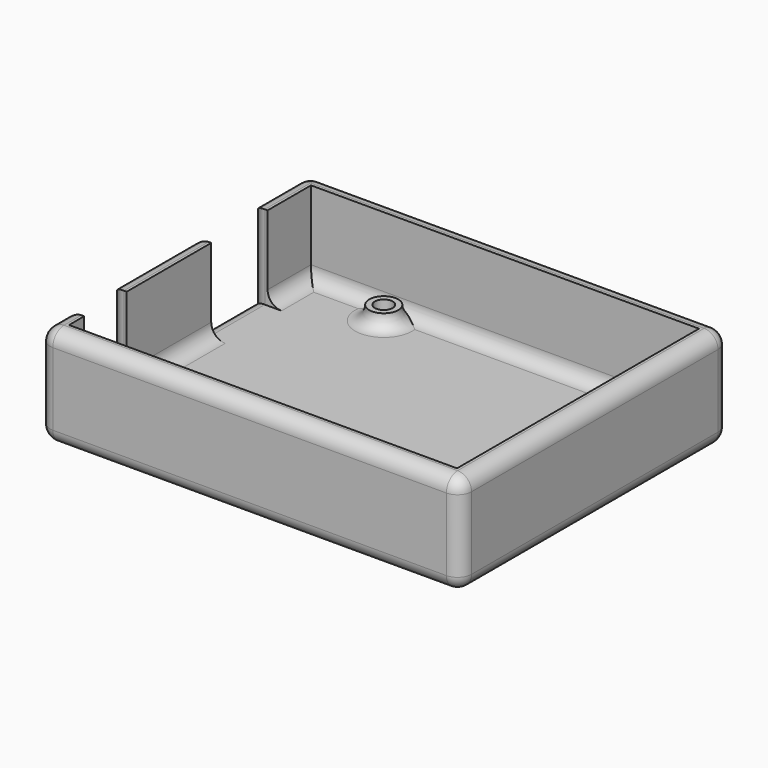
from build123d import *

# Parameters (mm, degrees)
F0_W          = 0.4
F0_H          = 0.3
F0_H_2        = 8.9
F0_W_2        = 9.5
F0_R          = 2.6
F0_W_3        = 10.3
F0_H_3        = 12
F0_W_4        = 3
F0_R_2        = 1.6
F0_H_4        = 18.9
F1_DEPTH      = 3
F2_DEPTH      = 15
F3_DEPTH      = 2.5
F4_T1_DEPTH   = 9.7
F4_T3_DEPTH   = 18.9
F4_T5_DEPTH   = 3.4
F4_T10_DEPTH  = 69.4
F4_S11_R      = 2.6
F4_T12_DEPTH  = 36
F4_T16_DEPTH  = 69.4
F4_S17_R      = 2.6
F4_T18_DEPTH  = 36
F4_T22_DEPTH  = 54.1
F4_S23_R      = 2.6
F4_T24_DEPTH  = 29
F4_S25_R      = 2.6
F4_T26_DEPTH  = 29
F4_T35_DEPTH  = 13
F4_T37_DEPTH  = 21.25
F4_T39_DEPTH  = 12.6
F4_T41_DEPTH  = 9.5
F4_T43_DEPTH  = 55.1
F4_T45_DEPTH  = 70.4
F4_T47_DEPTH  = 31.4
F4_T49_DEPTH  = 16.45
F4_T51_DEPTH  = 10.15
F4_S55_W      = 2.55
F4_S55_H      = 2.55
F4_T56_DEPTH  = 2.55
F4_S61_W      = 2.55
F4_S61_H      = 2.55
F4_T62_DEPTH  = 2.55
F4_S67_W      = 2.55
F4_S67_H      = 2.55
F4_T68_DEPTH  = 2.55
F4_S73_W      = 2.55
F4_S73_H      = 2.55
F4_T74_DEPTH  = 2.55
F4_S79_W      = 2.55
F4_S79_H      = 2.55
F4_T80_DEPTH  = 2.55
F4_S85_W      = 2.55
F4_S85_H      = 2.55
F4_T86_DEPTH  = 2.55
F4_S91_W      = 2.55
F4_S91_H      = 2.55
F4_T92_DEPTH  = 2.55
F4_S97_W      = 2.55
F4_S97_H      = 2.55
F4_T98_DEPTH  = 2.55
F4_T105_DEPTH = 15.75
F4_T109_DEPTH = 21.25
F4_T117_DEPTH = 18.85
F4_T121_DEPTH = 21.25
F4_T129_DEPTH = 21.25
F4_T134_DEPTH = 18.85
F4_T141_DEPTH = 21.25
F4_T146_DEPTH = 15.75


# Not quite as in the source:
# - a fillet or chamfer that OpenCascade refuses, or shapes differently, is made with other operations: its cross-section is extruded or revolved along the edge and cut away or added


with BuildPart() as f1:
    # F0 (on Top) → F1 (new body)
    with BuildSketch(Plane.XY):
        Polygon((-34.7, -27.05), (-34.7, -23.65), (-37.7, -23.65), (-37.7, -30.05), (37.7, -30.05), (37.7, 30.05), (-37.7, 30.05), (-37.7, 17.35), (-34.7, 17.35), (-34.7, 27.05), (34.7, 27.05), (34.7, -27.05), align=None)
        with Locations((-34.5, -14.3)):
            Rectangle(F0_W, F0_H)
        with Locations((-34.5, -18.9)):
            Rectangle(F0_W, F0_H_2)
        with Locations((-29.55, -18.9)):
            Rectangle(F0_W_2, F0_H_2)
        Polygon((-34.3, -26.65), (34.3, -26.65), (34.3, 26.65), (-34.3, 26.65), (-34.3, 17.35), (-23.7, 17.35), (-23.7, 4.75), (-34.3, 4.75), (-34.3, -14.15), (-24.5, -14.15), (-24.5, -23.65), (-34.3, -23.65), align=None)
        with Locations((-20.3, -23.85)):
            Circle(F0_R, mode=Mode.SUBTRACT)
        with Locations((31.6, -19.15)):
            Circle(F0_R, mode=Mode.SUBTRACT)
        with Locations((-19.2, 23.95)):
            Circle(F0_R, mode=Mode.SUBTRACT)
        with Locations((31.6, 8.75)):
            Circle(F0_R, mode=Mode.SUBTRACT)
        Polygon((34.3, 26.65), (34.3, -26.65), (-34.3, -26.65), (-34.3, -23.65), (-34.7, -23.65), (-34.7, -27.05), (34.7, -27.05), (34.7, 27.05), (-34.7, 27.05), (-34.7, 17.35), (-34.3, 17.35), (-34.3, 26.65), align=None)
        with Locations((-29.15, 11.05)):
            Rectangle(F0_W_3, F0_H_3)
        with Locations((-36.2, 11.05)):
            Rectangle(F0_W_4, F0_H_3)
        with Locations((-34.5, 11.05)):
            Rectangle(F0_W, F0_H_3)
        with Locations((-36.2, -18.9)):
            Rectangle(F0_W_4, F0_H_2)
        with Locations((-36.2, -14.3)):
            Rectangle(F0_W_4, F0_H)
        with Locations((-19.2, 23.95)):
            Circle(F0_R)
        with Locations((-19.2, 23.95)):
            Circle(F0_R_2, mode=Mode.SUBTRACT)
        with Locations((-20.3, -23.85)):
            Circle(F0_R)
        with Locations((-20.3, -23.85)):
            Circle(F0_R_2, mode=Mode.SUBTRACT)
        with Locations((31.6, -19.15)):
            Circle(F0_R)
        with Locations((31.6, -19.15)):
            Circle(F0_R_2, mode=Mode.SUBTRACT)
        with Locations((31.6, 8.75)):
            Circle(F0_R)
        with Locations((31.6, 8.75)):
            Circle(F0_R_2, mode=Mode.SUBTRACT)
        with Locations((-36.2, 4.9)):
            Rectangle(F0_W_4, F0_H)
        with Locations((-34.5, 4.9)):
            Rectangle(F0_W, F0_H)
        Polygon((-23.7, 17.35), (-34.3, 17.35), (-34.3, 17.05), (-24, 17.05), (-24, 5.05), (-34.3, 5.05), (-34.3, 4.75), (-23.7, 4.75), align=None)
        with Locations((-34.5, -4.7)):
            Rectangle(F0_W, F0_H_4)
        with Locations((-36.2, -4.7)):
            Rectangle(F0_W_4, F0_H_4)
        Polygon((-34.3, -23.35), (-34.3, -23.65), (-24.5, -23.65), (-24.5, -14.15), (-34.3, -14.15), (-34.3, -14.45), (-24.8, -14.45), (-24.8, -23.35), align=None)
        with Locations((-36.2, 17.2)):
            Rectangle(F0_W_4, F0_H)
        with Locations((-34.5, 17.2)):
            Rectangle(F0_W, F0_H)
        with Locations((-34.5, -23.5)):
            Rectangle(F0_W, F0_H)
        with Locations((-36.2, -23.5)):
            Rectangle(F0_W_4, F0_H)
    extrude(amount=-F1_DEPTH)

    # F0 (on Top) → F2 (join)
    with BuildSketch(Plane.XY):
        Polygon((-34.7, -27.05), (-34.7, -23.65), (-37.7, -23.65), (-37.7, -30.05), (37.7, -30.05), (37.7, 30.05), (-37.7, 30.05), (-37.7, 17.35), (-34.7, 17.35), (-34.7, 27.05), (34.7, 27.05), (34.7, -27.05), align=None)
        with Locations((-36.2, -4.7)):
            Rectangle(F0_W_4, F0_H_4)
    extrude(amount=F2_DEPTH)

    # F0 (on Top) → F3 (join)
    with BuildSketch(Plane.XY):
        with Locations((-20.3, -23.85)):
            Circle(F0_R)
        with Locations((-20.3, -23.85)):
            Circle(F0_R_2, mode=Mode.SUBTRACT)
        with Locations((-19.2, 23.95)):
            Circle(F0_R)
        with Locations((-19.2, 23.95)):
            Circle(F0_R_2, mode=Mode.SUBTRACT)
        with Locations((31.6, 8.75)):
            Circle(F0_R)
        with Locations((31.6, 8.75)):
            Circle(F0_R_2, mode=Mode.SUBTRACT)
        with Locations((31.6, -19.15)):
            Circle(F0_R)
        with Locations((31.6, -19.15)):
            Circle(F0_R_2, mode=Mode.SUBTRACT)
    extrude(amount=F3_DEPTH)

    # F4: fillet of radius 2.5 on 30 edges, made by hand

    # F4_s2 → F4_t1 (join)
    with BuildSketch(Plane.XZ.offset(-27.05)):
        with BuildLine():
            ThreePointArc((-34.7, 2.5), (-33.967766953, 0.732233047), (-32.2, 0))
            Line((-32.2, 0), (-34.7, 0))
            Line((-34.7, 0), (-34.7, 2.5))
        make_face()
    extrude(amount=F4_T1_DEPTH)

    # F4_s4 → F4_t3 (join)
    with BuildSketch(Plane.XZ.offset(-4.75)):
        with BuildLine():
            ThreePointArc((-32.2, 0), (-33.967766953, 0.732233047), (-34.7, 2.5))
            Line((-34.7, 2.5), (-34.7, 0))
            Line((-34.7, 0), (-32.2, 0))
        make_face()
    extrude(amount=F4_T3_DEPTH)

    # F4_s6 → F4_t5 (join)
    with BuildSketch(Plane.XZ.offset(23.65)):
        with BuildLine():
            ThreePointArc((-34.7, 2.5), (-33.967766953, 0.732233047), (-32.2, 0))
            Line((-32.2, 0), (-34.7, 0))
            Line((-34.7, 0), (-34.7, 2.5))
        make_face()
    extrude(amount=F4_T5_DEPTH)


with BuildPart() as f4_tool8:
    # F4_s9 → F4_t10 (new body)
    with BuildSketch(Plane.YZ.offset(-34.7)):
        with BuildLine():
            ThreePointArc((27.05, 2.5), (26.317766953, 0.732233047), (24.55, 0))
            Line((24.55, 0), (27.05, 0))
            Line((27.05, 0), (27.05, 2.5))
        make_face()
    extrude(amount=F4_T10_DEPTH)

    # F4_s11 → F4_t12 (cut, symmetric)
    with BuildSketch(Plane.XY.offset(1.2)):
        with Locations((-19.2, 23.95)):
            Circle(F4_S11_R)
    extrude(amount=F4_T12_DEPTH, both=True, mode=Mode.SUBTRACT)


with BuildPart() as f1_1:
    add(f1.part)

    # F4_t7: union F4_tool8
    add(f4_tool8.part)


with BuildPart() as f4_tool14:
    # F4_s15 → F4_t16 (new body)
    with BuildSketch(Plane.YZ.offset(34.7)):
        with BuildLine():
            ThreePointArc((-27.05, 2.5), (-26.317766953, 0.732233047), (-24.55, 0))
            Line((-24.55, 0), (-27.05, 0))
            Line((-27.05, 0), (-27.05, 2.5))
        make_face()
    extrude(amount=-F4_T16_DEPTH)

    # F4_s17 → F4_t18 (cut, symmetric)
    with BuildSketch(Plane.XY.offset(1.2)):
        with Locations((-20.3, -23.85)):
            Circle(F4_S17_R)
    extrude(amount=F4_T18_DEPTH, both=True, mode=Mode.SUBTRACT)


with BuildPart() as f1_2:
    add(f1_1.part)

    # F4_t13: union F4_tool14
    add(f4_tool14.part)


with BuildPart() as f4_tool20:
    # F4_s21 → F4_t22 (new body)
    with BuildSketch(Plane.XZ.offset(-27.05)):
        with BuildLine():
            ThreePointArc((34.7, 2.5), (33.967766953, 0.732233047), (32.2, 0))
            Line((32.2, 0), (34.7, 0))
            Line((34.7, 0), (34.7, 2.5))
        make_face()
    extrude(amount=F4_T22_DEPTH)

    # F4_s23 → F4_t24 (cut, symmetric)
    with BuildSketch(Plane.XY.offset(1.2)):
        with Locations((31.6, -19.15)):
            Circle(F4_S23_R)
    extrude(amount=F4_T24_DEPTH, both=True, mode=Mode.SUBTRACT)

    # F4_s25 → F4_t26 (cut, symmetric)
    with BuildSketch(Plane.XY.offset(1.2)):
        with Locations((31.6, 8.75)):
            Circle(F4_S25_R)
    extrude(amount=F4_T26_DEPTH, both=True, mode=Mode.SUBTRACT)


with BuildPart() as f1_3:
    add(f1_2.part)

    # F4_t19: union F4_tool20
    add(f4_tool20.part)

    # F4_s27 → F4_t28 (revolve)
    with BuildSketch(Plane.XZ.offset(-8.75)):
        with BuildLine():
            ThreePointArc((36.7, 0), (34.932233047, 0.732233047), (34.2, 2.5))
            Line((34.2, 2.5), (34.2, 0))
            Line((34.2, 0), (36.7, 0))
        make_face()
    revolve(axis=Axis((31.6, 8.75, 0), (0, 0, 1)))

    # F4_s29 → F4_t30 (revolve)
    with BuildSketch(Plane.XZ.offset(19.15)):
        with BuildLine():
            ThreePointArc((36.7, 0), (34.932233047, 0.732233047), (34.2, 2.5))
            Line((34.2, 2.5), (34.2, 0))
            Line((34.2, 0), (36.7, 0))
        make_face()
    revolve(axis=Axis((31.6, -19.15, 0), (0, 0, 1)))

    # F4_s31 → F4_t32 (revolve)
    with BuildSketch(Plane.XZ.offset(23.85)):
        with BuildLine():
            ThreePointArc((-15.2, 0), (-16.967766953, 0.732233047), (-17.7, 2.5))
            Line((-17.7, 2.5), (-17.7, 0))
            Line((-17.7, 0), (-15.2, 0))
        make_face()
    revolve(axis=Axis((-20.3, -23.85, 0), (0, 0, 1)))

    # F4_s33 → F4_t34 (revolve)
    with BuildSketch(Plane.XZ.offset(-23.95)):
        with BuildLine():
            ThreePointArc((-14.1, 0), (-15.867766953, 0.732233047), (-16.6, 2.5))
            Line((-16.6, 2.5), (-16.6, 0))
            Line((-16.6, 0), (-14.1, 0))
        make_face()
    revolve(axis=Axis((-19.2, 23.95, 0), (0, 0, 1)))

    # F4_s36 → F4_t35 (cut)
    with BuildSketch(Plane.XY.offset(-0.5)):
        with BuildLine():
            ThreePointArc((35.2, -30.05), (36.967766953, -29.317766953), (37.7, -27.55))
            Line((37.7, -27.55), (37.7, -30.05))
            Line((37.7, -30.05), (35.2, -30.05))
        make_face()
        with BuildLine():
            ThreePointArc((37.7, 27.55), (36.967766953, 29.317766953), (35.2, 30.05))
            Line((35.2, 30.05), (37.7, 30.05))
            Line((37.7, 30.05), (37.7, 27.55))
        make_face()
        with BuildLine():
            ThreePointArc((-37.7, 27.55), (-36.967766953, 29.317766953), (-35.2, 30.05))
            Line((-35.2, 30.05), (-37.7, 30.05))
            Line((-37.7, 30.05), (-37.7, 27.55))
        make_face()
        with BuildLine():
            ThreePointArc((-35.2, -30.05), (-36.967766953, -29.317766953), (-37.7, -27.55))
            Line((-37.7, -27.55), (-37.7, -30.05))
            Line((-37.7, -30.05), (-35.2, -30.05))
        make_face()
    extrude(amount=F4_T35_DEPTH, mode=Mode.SUBTRACT)

    # F4_s38 → F4_t37 (cut)
    with BuildSketch(Plane.XY):
        with BuildLine():
            ThreePointArc((-37.7, -11.65), (-36.967766953, -13.417766953), (-35.2, -14.15))
            Line((-35.2, -14.15), (-37.7, -14.15))
            Line((-37.7, -14.15), (-37.7, -11.65))
        make_face()
        with BuildLine():
            ThreePointArc((-37.7, 19.85), (-36.967766953, 18.082233047), (-35.2, 17.35))
            Line((-35.2, 17.35), (-37.7, 17.35))
            Line((-37.7, 17.35), (-37.7, 19.85))
        make_face()
        with BuildLine():
            ThreePointArc((-37.7, 2.25), (-36.967766953, 4.017766953), (-35.2, 4.75))
            Line((-35.2, 4.75), (-37.7, 4.75))
            Line((-37.7, 4.75), (-37.7, 2.25))
        make_face()
        with BuildLine():
            ThreePointArc((-37.7, -26.15), (-36.967766953, -24.382233047), (-35.2, -23.65))
            Line((-35.2, -23.65), (-37.7, -23.65))
            Line((-37.7, -23.65), (-37.7, -26.15))
        make_face()
    extrude(amount=F4_T37_DEPTH, mode=Mode.SUBTRACT)

    # F4_s40 → F4_t39 (cut)
    with BuildSketch(Plane.XZ.offset(-17.35)):
        with BuildLine():
            ThreePointArc((-37.7, -2.5), (-36.967766953, -0.732233047), (-35.2, 0))
            Line((-35.2, 0), (-37.7, 0))
            Line((-37.7, 0), (-37.7, -2.5))
        make_face()
    extrude(amount=F4_T39_DEPTH, mode=Mode.SUBTRACT)

    # F4_s42 → F4_t41 (cut)
    with BuildSketch(Plane.XZ.offset(14.15)):
        with BuildLine():
            ThreePointArc((-37.7, -2.5), (-36.967766953, -0.732233047), (-35.2, 0))
            Line((-35.2, 0), (-37.7, 0))
            Line((-37.7, 0), (-37.7, -2.5))
        make_face()
    extrude(amount=F4_T41_DEPTH, mode=Mode.SUBTRACT)

    # F4_s44 → F4_t43 (cut)
    with BuildSketch(Plane.XZ.offset(-27.55)):
        with BuildLine():
            ThreePointArc((35.2, -3), (36.967766953, -2.267766953), (37.7, -0.5))
            Line((37.7, -0.5), (37.7, -3))
            Line((37.7, -3), (35.2, -3))
        make_face()
        with BuildLine():
            ThreePointArc((-35.2, -3), (-36.967766953, -2.267766953), (-37.7, -0.5))
            Line((-37.7, -0.5), (-37.7, -3))
            Line((-37.7, -3), (-35.2, -3))
        make_face()
        with BuildLine():
            ThreePointArc((37.7, 12.5), (36.967766953, 14.267766953), (35.2, 15))
            Line((35.2, 15), (37.7, 15))
            Line((37.7, 15), (37.7, 12.5))
        make_face()
    extrude(amount=F4_T43_DEPTH, mode=Mode.SUBTRACT)

    # F4_s46 → F4_t45 (cut)
    with BuildSketch(Plane.YZ.offset(-35.2)):
        with BuildLine():
            ThreePointArc((27.55, -3), (29.317766953, -2.267766953), (30.05, -0.5))
            Line((30.05, -0.5), (30.05, -3))
            Line((30.05, -3), (27.55, -3))
        make_face()
        with BuildLine():
            ThreePointArc((-30.05, -0.5), (-29.317766953, -2.267766953), (-27.55, -3))
            Line((-27.55, -3), (-30.05, -3))
            Line((-30.05, -3), (-30.05, -0.5))
        make_face()
        with BuildLine():
            ThreePointArc((27.55, 15), (29.317766953, 14.267766953), (30.05, 12.5))
            Line((30.05, 12.5), (30.05, 15))
            Line((30.05, 15), (27.55, 15))
        make_face()
        with BuildLine():
            ThreePointArc((-30.05, 12.5), (-29.317766953, 14.267766953), (-27.55, 15))
            Line((-27.55, 15), (-30.05, 15))
            Line((-30.05, 15), (-30.05, 12.5))
        make_face()
    extrude(amount=F4_T45_DEPTH, mode=Mode.SUBTRACT)

    # F4_s48 → F4_t47 (cut)
    with BuildSketch(Plane.XZ.offset(-11)):
        with BuildLine():
            ThreePointArc((-37.7, 12.5), (-36.967766953, 14.267766953), (-35.2, 15))
            Line((-35.2, 15), (-37.7, 15))
            Line((-37.7, 15), (-37.7, 12.5))
        make_face()
    extrude(amount=F4_T47_DEPTH, mode=Mode.SUBTRACT)

    # F4_s50 → F4_t49 (cut)
    with BuildSketch(Plane.XZ.offset(-27.55)):
        with BuildLine():
            ThreePointArc((-35.2, 15), (-36.967766953, 14.267766953), (-37.7, 12.5))
            Line((-37.7, 12.5), (-37.7, 15))
            Line((-37.7, 15), (-35.2, 15))
        make_face()
    extrude(amount=F4_T49_DEPTH, mode=Mode.SUBTRACT)

    # F4_s52 → F4_t51 (cut)
    with BuildSketch(Plane.XZ.offset(17.4)):
        with BuildLine():
            ThreePointArc((-35.2, 15), (-36.967766953, 14.267766953), (-37.7, 12.5))
            Line((-37.7, 12.5), (-37.7, 15))
            Line((-37.7, 15), (-35.2, 15))
        make_face()
    extrude(amount=F4_T51_DEPTH, mode=Mode.SUBTRACT)


with BuildPart() as f4_tool54:
    # F4_s55 → F4_t56 (new body)
    with BuildSketch(Plane.XZ.offset(27.55)):
        with Locations((36.475, -1.775)):
            Rectangle(F4_S55_W, F4_S55_H)
    extrude(amount=F4_T56_DEPTH)

    # F4_s57 → F4_t58 (revolve, cut)
    with BuildSketch(Plane(origin=(35.2, -27.55, -0.5), x_dir=(-0.7071067812, 0, 0.7071067812), z_dir=(0.7071067812, 0, 0.7071067812))):
        with BuildLine():
            ThreePointArc((0, -2.5), (2.5, 0), (0, 2.5))
            Line((0, 2.5), (0, -2.5))
        make_face()
    revolve(axis=Axis((35.2, -27.55, -0.5), (0, -1, 0)), mode=Mode.SUBTRACT)


with BuildPart() as f1_4:
    add(f1_3.part)

    # F4_t53: cut F4_tool54
    add(f4_tool54.part, mode=Mode.SUBTRACT)


with BuildPart() as f4_tool60:
    # F4_s61 → F4_t62 (new body)
    with BuildSketch(Plane.XZ.offset(27.55)):
        with Locations((36.475, 13.775)):
            Rectangle(F4_S61_W, F4_S61_H)
    extrude(amount=F4_T62_DEPTH)

    # F4_s63 → F4_t64 (revolve, cut)
    with BuildSketch(Plane(origin=(35.2, -27.55, 12.5), x_dir=(-0.7071067812, 0, -0.7071067812), z_dir=(-0.7071067812, 0, 0.7071067812))):
        with BuildLine():
            ThreePointArc((0, -2.5), (2.5, 0), (0, 2.5))
            Line((0, 2.5), (0, -2.5))
        make_face()
    revolve(axis=Axis((35.2, -27.55, 12.5), (0, -1, 0)), mode=Mode.SUBTRACT)


with BuildPart() as f1_5:
    add(f1_4.part)

    # F4_t59: cut F4_tool60
    add(f4_tool60.part, mode=Mode.SUBTRACT)


with BuildPart() as f4_tool66:
    # F4_s67 → F4_t68 (new body)
    with BuildSketch(Plane.XY.offset(-0.5)):
        with Locations((36.475, 28.825)):
            Rectangle(F4_S67_W, F4_S67_H)
    extrude(amount=-F4_T68_DEPTH)

    # F4_s69 → F4_t70 (revolve, cut)
    with BuildSketch(Plane(origin=(35.2, 27.55, -0.5), x_dir=(-0.7071067812, -0.7071067812, 0), z_dir=(0.7071067812, -0.7071067812, 0))):
        with BuildLine():
            ThreePointArc((0, -2.5), (2.5, 0), (0, 2.5))
            Line((0, 2.5), (0, -2.5))
        make_face()
    revolve(axis=Axis((35.2, 27.55, -0.5), (0, 0, -1)), mode=Mode.SUBTRACT)


with BuildPart() as f1_6:
    add(f1_5.part)

    # F4_t65: cut F4_tool66
    add(f4_tool66.part, mode=Mode.SUBTRACT)


with BuildPart() as f4_tool72:
    # F4_s73 → F4_t74 (new body)
    with BuildSketch(Plane.YZ.offset(35.2)):
        with Locations((28.825, 13.775)):
            Rectangle(F4_S73_W, F4_S73_H)
    extrude(amount=F4_T74_DEPTH)

    # F4_s75 → F4_t76 (revolve, cut)
    with BuildSketch(Plane(origin=(35.2, 27.55, 12.5), x_dir=(0, -0.7071067812, -0.7071067812), z_dir=(0, -0.7071067812, 0.7071067812))):
        with BuildLine():
            ThreePointArc((0, -2.5), (2.5, 0), (0, 2.5))
            Line((0, 2.5), (0, -2.5))
        make_face()
    revolve(axis=Axis((35.2, 27.55, 12.5), (1, 0, 0)), mode=Mode.SUBTRACT)


with BuildPart() as f1_7:
    add(f1_6.part)

    # F4_t71: cut F4_tool72
    add(f4_tool72.part, mode=Mode.SUBTRACT)


with BuildPart() as f4_tool78:
    # F4_s79 → F4_t80 (new body)
    with BuildSketch(Plane.XY.offset(12.5)):
        with Locations((-36.475, 28.825)):
            Rectangle(F4_S79_W, F4_S79_H)
    extrude(amount=F4_T80_DEPTH)

    # F4_s81 → F4_t82 (revolve, cut)
    with BuildSketch(Plane(origin=(-35.2, 27.55, 12.5), x_dir=(0.7071067812, -0.7071067812, 0), z_dir=(-0.7071067812, -0.7071067812, 0))):
        with BuildLine():
            ThreePointArc((0, -2.5), (2.5, 0), (0, 2.5))
            Line((0, 2.5), (0, -2.5))
        make_face()
    revolve(axis=Axis((-35.2, 27.55, 12.5), (0, 0, 1)), mode=Mode.SUBTRACT)


with BuildPart() as f1_8:
    add(f1_7.part)

    # F4_t77: cut F4_tool78
    add(f4_tool78.part, mode=Mode.SUBTRACT)


with BuildPart() as f4_tool84:
    # F4_s85 → F4_t86 (new body)
    with BuildSketch(Plane.XY.offset(-0.5)):
        with Locations((-36.475, 28.825)):
            Rectangle(F4_S85_W, F4_S85_H)
    extrude(amount=-F4_T86_DEPTH)

    # F4_s87 → F4_t88 (revolve, cut)
    with BuildSketch(Plane(origin=(-35.2, 27.55, -0.5), x_dir=(0.7071067812, -0.7071067812, 0), z_dir=(0.7071067812, 0.7071067812, 0))):
        with BuildLine():
            ThreePointArc((0, -2.5), (2.5, 0), (0, 2.5))
            Line((0, 2.5), (0, -2.5))
        make_face()
    revolve(axis=Axis((-35.2, 27.55, -0.5), (0, 0, -1)), mode=Mode.SUBTRACT)


with BuildPart() as f1_9:
    add(f1_8.part)

    # F4_t83: cut F4_tool84
    add(f4_tool84.part, mode=Mode.SUBTRACT)


with BuildPart() as f4_tool90:
    # F4_s91 → F4_t92 (new body)
    with BuildSketch(Plane.XZ.offset(27.55)):
        with Locations((-36.475, 13.775)):
            Rectangle(F4_S91_W, F4_S91_H)
    extrude(amount=F4_T92_DEPTH)

    # F4_s93 → F4_t94 (revolve, cut)
    with BuildSketch(Plane(origin=(-35.2, -27.55, 12.5), x_dir=(0.7071067812, 0, -0.7071067812), z_dir=(-0.7071067812, 0, -0.7071067812))):
        with BuildLine():
            ThreePointArc((0, -2.5), (2.5, 0), (0, 2.5))
            Line((0, 2.5), (0, -2.5))
        make_face()
    revolve(axis=Axis((-35.2, -27.55, 12.5), (0, -1, 0)), mode=Mode.SUBTRACT)


with BuildPart() as f1_10:
    add(f1_9.part)

    # F4_t89: cut F4_tool90
    add(f4_tool90.part, mode=Mode.SUBTRACT)


with BuildPart() as f4_tool96:
    # F4_s97 → F4_t98 (new body)
    with BuildSketch(Plane.XZ.offset(27.55)):
        with Locations((-36.475, -1.775)):
            Rectangle(F4_S97_W, F4_S97_H)
    extrude(amount=F4_T98_DEPTH)

    # F4_s99 → F4_t100 (revolve, cut)
    with BuildSketch(Plane(origin=(-35.2, -27.55, -0.5), x_dir=(0.7071067812, 0, 0.7071067812), z_dir=(0.7071067812, 0, -0.7071067812))):
        with BuildLine():
            ThreePointArc((0, -2.5), (2.5, 0), (0, 2.5))
            Line((0, 2.5), (0, -2.5))
        make_face()
    revolve(axis=Axis((-35.2, -27.55, -0.5), (0, -1, 0)), mode=Mode.SUBTRACT)


with BuildPart() as f1_11:
    add(f1_10.part)

    # F4_t95: cut F4_tool96
    add(f4_tool96.part, mode=Mode.SUBTRACT)


with BuildPart() as f4_tool103:
    # F4_s104 → F4_t105 (new body)
    with BuildSketch(Plane.XZ.offset(7.9)):
        with BuildLine():
            ThreePointArc((-37.7, -2.5), (-36.967766953, -0.732233047), (-35.2, 0))
            Line((-35.2, 0), (-37.7, 0))
            Line((-37.7, 0), (-37.7, -2.5))
        make_face()
    extrude(amount=F4_T105_DEPTH)

    split(bisect_by=Plane.XZ.offset(14.15), keep=Keep.BOTTOM)


with BuildPart() as f4_tool107:
    # F4_s108 → F4_t109 (new body)
    with BuildSketch(Plane.XY.offset(-6.25)):
        with BuildLine():
            ThreePointArc((-37.7, -11.65), (-36.967766953, -13.417766953), (-35.2, -14.15))
            Line((-35.2, -14.15), (-37.7, -14.15))
            Line((-37.7, -14.15), (-37.7, -11.65))
        make_face()
    extrude(amount=F4_T109_DEPTH)

    split(bisect_by=Plane.XY.offset(-3), keep=Keep.TOP)

    split(bisect_by=Plane.XY, keep=Keep.BOTTOM)


with BuildPart() as f4_tool103_1:
    add(f4_tool103.part)

    # F4_t112: intersect F4_tool107
    add(f4_tool107.part, mode=Mode.INTERSECT)


with BuildPart() as f1_12:
    add(f1_11.part)

    # F4_t101: cut F4_tool103
    add(f4_tool103_1.part, mode=Mode.SUBTRACT)


with BuildPart() as f4_tool115:
    # F4_s116 → F4_t117 (new body)
    with BuildSketch(Plane.XZ.offset(-23.6)):
        with BuildLine():
            ThreePointArc((-37.7, -2.5), (-36.967766953, -0.732233047), (-35.2, 0))
            Line((-35.2, 0), (-37.7, 0))
            Line((-37.7, 0), (-37.7, -2.5))
        make_face()
    extrude(amount=F4_T117_DEPTH)

    split(bisect_by=Plane.XZ.offset(-17.35), keep=Keep.BOTTOM)


with BuildPart() as f4_tool119:
    # F4_s120 → F4_t121 (new body)
    with BuildSketch(Plane.XY.offset(-6.25)):
        with BuildLine():
            ThreePointArc((-37.7, 19.85), (-36.967766953, 18.082233047), (-35.2, 17.35))
            Line((-35.2, 17.35), (-37.7, 17.35))
            Line((-37.7, 17.35), (-37.7, 19.85))
        make_face()
    extrude(amount=F4_T121_DEPTH)

    split(bisect_by=Plane.XY.offset(-3), keep=Keep.TOP)

    split(bisect_by=Plane.XY, keep=Keep.BOTTOM)


with BuildPart() as f4_tool115_1:
    add(f4_tool115.part)

    # F4_t124: intersect F4_tool119
    add(f4_tool119.part, mode=Mode.INTERSECT)


with BuildPart() as f1_13:
    add(f1_12.part)

    # F4_t113: cut F4_tool115
    add(f4_tool115_1.part, mode=Mode.SUBTRACT)


with BuildPart() as f4_tool127:
    # F4_s128 → F4_t129 (new body)
    with BuildSketch(Plane.XY.offset(-6.25)):
        with BuildLine():
            ThreePointArc((-37.7, 2.25), (-36.967766953, 4.017766953), (-35.2, 4.75))
            Line((-35.2, 4.75), (-37.7, 4.75))
            Line((-37.7, 4.75), (-37.7, 2.25))
        make_face()
    extrude(amount=F4_T129_DEPTH)

    split(bisect_by=Plane.XY.offset(-3), keep=Keep.TOP)

    split(bisect_by=Plane.XY, keep=Keep.BOTTOM)


with BuildPart() as f4_tool132:
    # F4_s133 → F4_t134 (new body)
    with BuildSketch(Plane.XZ.offset(-17.35)):
        with BuildLine():
            ThreePointArc((-37.7, -2.5), (-36.967766953, -0.732233047), (-35.2, 0))
            Line((-35.2, 0), (-37.7, 0))
            Line((-37.7, 0), (-37.7, -2.5))
        make_face()
    extrude(amount=F4_T134_DEPTH)

    split(bisect_by=Plane.XZ.offset(-4.75), keep=Keep.TOP)


with BuildPart() as f4_tool127_1:
    add(f4_tool127.part)

    # F4_t136: intersect F4_tool132
    add(f4_tool132.part, mode=Mode.INTERSECT)


with BuildPart() as f1_14:
    add(f1_13.part)

    # F4_t125: cut F4_tool127
    add(f4_tool127_1.part, mode=Mode.SUBTRACT)


with BuildPart() as f4_tool139:
    # F4_s140 → F4_t141 (new body)
    with BuildSketch(Plane.XY.offset(-6.25)):
        with BuildLine():
            ThreePointArc((-37.7, -26.15), (-36.967766953, -24.382233047), (-35.2, -23.65))
            Line((-35.2, -23.65), (-37.7, -23.65))
            Line((-37.7, -23.65), (-37.7, -26.15))
        make_face()
    extrude(amount=F4_T141_DEPTH)

    split(bisect_by=Plane.XY.offset(-3), keep=Keep.TOP)

    split(bisect_by=Plane.XY, keep=Keep.BOTTOM)


with BuildPart() as f4_tool144:
    # F4_s145 → F4_t146 (new body)
    with BuildSketch(Plane.XZ.offset(14.15)):
        with BuildLine():
            ThreePointArc((-37.7, -2.5), (-36.967766953, -0.732233047), (-35.2, 0))
            Line((-35.2, 0), (-37.7, 0))
            Line((-37.7, 0), (-37.7, -2.5))
        make_face()
    extrude(amount=F4_T146_DEPTH)

    split(bisect_by=Plane.XZ.offset(23.65), keep=Keep.TOP)


with BuildPart() as f4_tool139_1:
    add(f4_tool139.part)

    # F4_t148: intersect F4_tool144
    add(f4_tool144.part, mode=Mode.INTERSECT)


with BuildPart() as f1_15:
    add(f1_14.part)

    # F4_t137: cut F4_tool139
    add(f4_tool139_1.part, mode=Mode.SUBTRACT)


solid = f1_15.part
